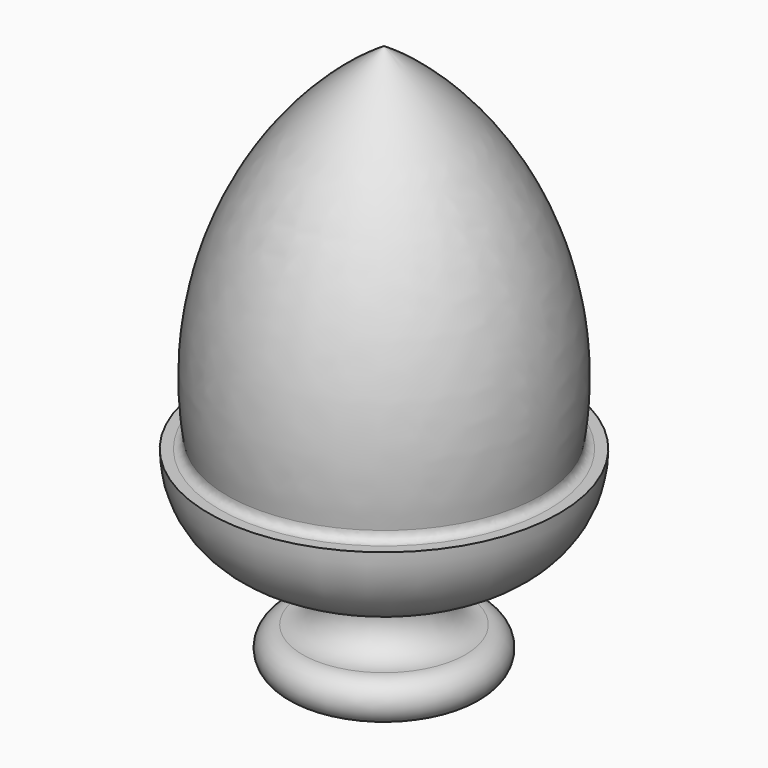
from build123d import *

# Parameters (mm, degrees)
F0_W     = 203.2
F0_H     = 203.2
F1_DEPTH = 17.78
F4_R     = 5.08
F5_W     = 203.2
F5_H     = 203.2
F6_DEPTH = 19


# Not quite as in the source:
# - a feature names something its author has since deleted; it is built from what else it names


with BuildPart() as f1:
    # F0 (on Top) → F1 (new body)
    with BuildSketch(Plane.XY):
        Rectangle(F0_W, F0_H)
    extrude(amount=F1_DEPTH)

    # F2 (on Front) → F3 (revolve)
    with BuildSketch(Plane.XZ):
        with BuildLine():
            Line((0, 360.68), (0, 17.78))
            Line((0, 17.78), (50.8, 17.78))
            ThreePointArc((50.8, 17.78), (63.5, 30.48), (50.8, 43.18))
            ThreePointArc((50.8, 43.18), (31.75, 62.23), (50.8, 81.28))
            ThreePointArc((50.8, 81.28), (92.1091781569, 98.3908218431), (109.22, 139.7))
            Line((109.22, 139.7), (96.52, 139.7))
            ThreePointArc((96.52, 139.7), (82.2548109307, 265.0383082226), (0, 360.68))
        make_face()
    revolve(axis=Axis((0, 0, 189.23), (0, 0, 1)))

    # F4
    f4_edges = [f1.edges().sort_by_distance(p)[0] for p in [
        (-96.52, 0, 139.7),
    ]]
    fillet(f4_edges, radius=F4_R)

    # F5 (on face) → F6 (cut)
    with BuildSketch(Plane(origin=(0, 0, 0), x_dir=(1, 0, 0), z_dir=(0, 0, -1))):
        Rectangle(F5_W, F5_H)
    extrude(amount=-F6_DEPTH, mode=Mode.SUBTRACT)


solid = f1.part
